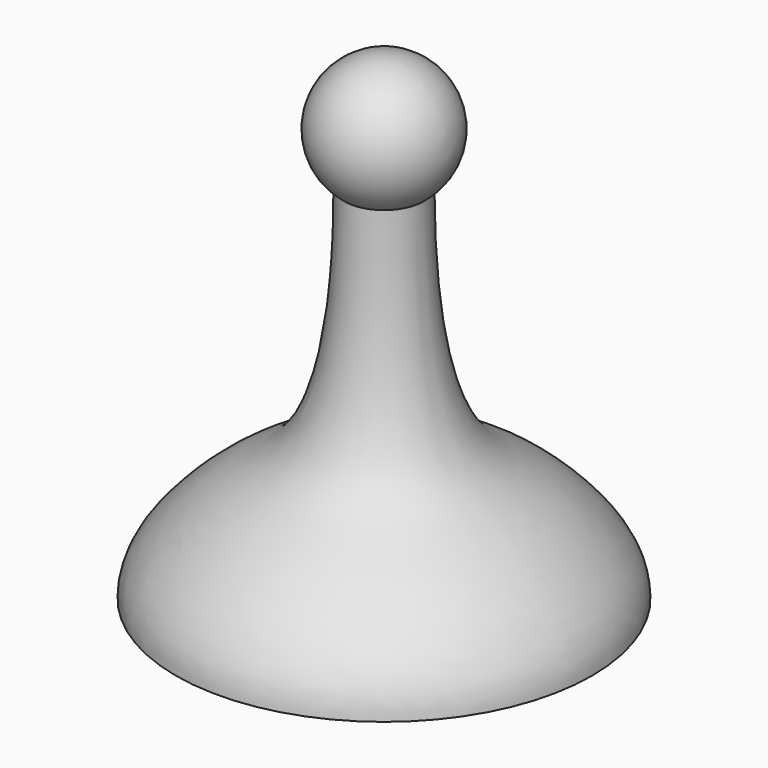
from build123d import *


with BuildPart() as f1:
    # F0 (on Front) → F1 (revolve)
    with BuildSketch(Plane.XZ):
        with BuildLine():
            add(Edge.make_bspline(
                [(2.0955, 19.2567927953), (2.0955, 14.1767927953), (2.9343024721, 7.4659610748), (7.0297915521, 5.4753950855), (9.6092095913, 3.303995323), (11.049, 1.27), (11.049, 0)],
                knots=[0, 0, 0, 0, 0.3769154067, 0.5916140053, 0.7930033614, 1, 1, 1, 1], degree=3))
            ThreePointArc((2.0955, 19.2567927953), (3.2453857633, 23.0780285667), (0, 25.4))
            Line((0, 25.4), (0, 0))
            Line((0, 0), (11.049, 0))
        make_face()
    revolve(axis=Axis((0, 0, 12.7), (0, 0, 1)))


solid = f1.part
